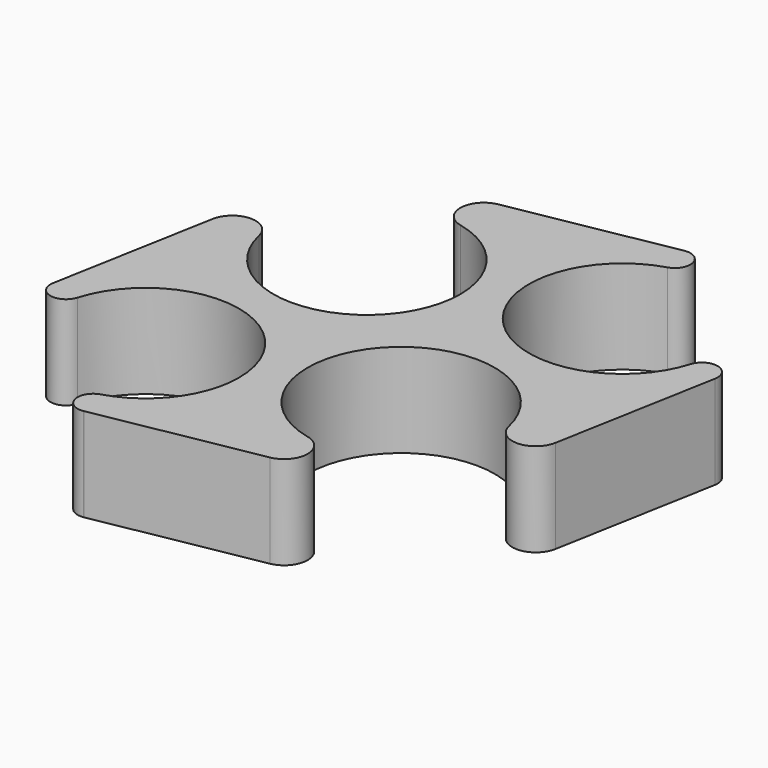
from build123d import *

# Parameters (mm, degrees)
F1_DEPTH    = 3
F2_T1_DEPTH = 13.3236108094
F2_T3_DEPTH = 16.5787171724
F3_F1_R     = 0.5
F3_F2_R     = 0.5
F3_F3_R     = 0.5
F3_F4_R     = 0.5
F4_R        = 0.75


# Not quite as in the source:
# - a fillet or chamfer that OpenCascade refuses, or shapes differently, is made with other operations: its cross-section is extruded or revolved along the edge and cut away or added


with BuildPart() as f1:
    # F0 (on Top) → F1 (new body)
    with BuildSketch(Plane.XY):
        with BuildLine():
            ThreePointArc((7.0690778624, 5.27606043), (7.204423259, 4.770944533), (7.25, 4.25))
            ThreePointArc((7.25, 4.25), (1.7925438671, 2.5292706909), (5.27606043, 7.0690778624))
            Line((5.27606043, 7.0690778624), (5.8261142664, 8.5803383574))
            Line((5.8261142664, 8.5803383574), (-4.2080450169, 6.7559457605))
            Line((-4.2080450169, 6.7559457605), (-3.77606043, 5.5690778624))
            ThreePointArc((-3.77606043, 5.5690778624), (-1.0292706909, 5.2074561329), (0.25, 2.75))
            ThreePointArc((0.25, 2.75), (-3.270944533, -0.204423259), (-5.5690778624, 3.77606043))
            Line((-5.5690778624, 3.77606043), (-6.7559457605, 4.2080450169))
            Line((-6.7559457605, 4.2080450169), (-8.5803383574, -5.8261142664))
            Line((-8.5803383574, -5.8261142664), (-7.0690778624, -5.27606043))
            ThreePointArc((-7.0690778624, -5.27606043), (-4.770944533, -1.295576741), (-1.25, -4.25))
            ThreePointArc((-1.25, -4.25), (-2.5292706909, -6.7074561329), (-5.27606043, -7.0690778624))
            Line((-5.27606043, -7.0690778624), (-5.8261142664, -8.5803383574))
            Line((-5.8261142664, -8.5803383574), (4.2080450169, -6.7559457605))
            Line((4.2080450169, -6.7559457605), (3.77606043, -5.5690778624))
            ThreePointArc((3.77606043, -5.5690778624), (0.2925438671, -1.0292706909), (5.75, -2.75))
            ThreePointArc((5.75, -2.75), (5.704423259, -3.270944533), (5.5690778624, -3.77606043))
            Line((5.5690778624, -3.77606043), (6.7559457605, -4.2080450169))
            Line((6.7559457605, -4.2080450169), (8.5803383574, 5.8261142664))
            Line((8.5803383574, 5.8261142664), (7.0690778624, 5.27606043))
        make_face()
    extrude(amount=F1_DEPTH)

    # F2: fillet of radius 2 on 8 edges, made by hand

    # F2_s2 → F2_t1 (cut)
    with BuildSketch(Plane.XY.offset(-5.1618054047)):
        with BuildLine():
            ThreePointArc((7.1252944891, -2.1766270091), (6.5910015424, -3.2135711792), (5.5690778624, -3.77606043))
            Line((5.5690778624, -3.77606043), (6.7559457605, -4.2080450169))
            Line((6.7559457605, -4.2080450169), (7.1252944891, -2.1766270091))
        make_face()
        with BuildLine():
            ThreePointArc((2.1766270091, -7.1252944891), (3.2135711792, -6.5910015424), (3.77606043, -5.5690778624))
            Line((3.77606043, -5.5690778624), (4.2080450169, -6.7559457605))
            Line((4.2080450169, -6.7559457605), (2.1766270091, -7.1252944891))
        make_face()
        with BuildLine():
            ThreePointArc((-3.77606043, 5.5690778624), (-3.2135711792, 6.5910015424), (-2.1766270091, 7.1252944891))
            Line((-2.1766270091, 7.1252944891), (-4.2080450169, 6.7559457605))
            Line((-4.2080450169, 6.7559457605), (-3.77606043, 5.5690778624))
        make_face()
        with BuildLine():
            ThreePointArc((-7.1252944891, 2.1766270091), (-6.5910015424, 3.2135711792), (-5.5690778624, 3.77606043))
            Line((-5.5690778624, 3.77606043), (-6.7559457605, 4.2080450169))
            Line((-6.7559457605, 4.2080450169), (-7.1252944891, 2.1766270091))
        make_face()
    extrude(amount=F2_T1_DEPTH, mode=Mode.SUBTRACT)

    # F2_s4 → F2_t3 (cut)
    with BuildSketch(Plane.XY.offset(-6.7893585862)):
        with BuildLine():
            ThreePointArc((7.0690778624, 5.27606043), (7.9275306923, 4.382198961), (8.0945314031, 3.1541760177))
            Line((8.0945314031, 3.1541760177), (8.5803383574, 5.8261142664))
            Line((8.5803383574, 5.8261142664), (7.0690778624, 5.27606043))
        make_face()
        with BuildLine():
            ThreePointArc((3.1541760177, 8.0945314031), (4.382198961, 7.9275306923), (5.27606043, 7.0690778624))
            Line((5.27606043, 7.0690778624), (5.8261142664, 8.5803383574))
            Line((5.8261142664, 8.5803383574), (3.1541760177, 8.0945314031))
        make_face()
        with BuildLine():
            ThreePointArc((-7.0690778624, -5.27606043), (-7.9275306923, -4.382198961), (-8.0945314031, -3.1541760177))
            Line((-8.0945314031, -3.1541760177), (-8.5803383574, -5.8261142664))
            Line((-8.5803383574, -5.8261142664), (-7.0690778624, -5.27606043))
        make_face()
        with BuildLine():
            ThreePointArc((-3.1541760177, -8.0945314031), (-4.382198961, -7.9275306923), (-5.27606043, -7.0690778624))
            Line((-5.27606043, -7.0690778624), (-5.8261142664, -8.5803383574))
            Line((-5.8261142664, -8.5803383574), (-3.1541760177, -8.0945314031))
        make_face()
    extrude(amount=F2_T3_DEPTH, mode=Mode.SUBTRACT)

    # F3: fillet of radius 0.5 on 4 edges, made by hand

    # F3_f1
    f3_f1_edges = [f1.edges().sort_by_distance(p)[0] for p in [
        (-5.27606043, -7.0690778624, 1.5),
    ]]
    fillet(f3_f1_edges, radius=F3_F1_R)

    # F3_f2
    f3_f2_edges = [f1.edges().sort_by_distance(p)[0] for p in [
        (-7.0690778624, -5.27606043, 1.5),
    ]]
    fillet(f3_f2_edges, radius=F3_F2_R)

    # F3_f3
    f3_f3_edges = [f1.edges().sort_by_distance(p)[0] for p in [
        (5.27606043, 7.0690778624, 1.5),
    ]]
    fillet(f3_f3_edges, radius=F3_F3_R)

    # F3_f4
    f3_f4_edges = [f1.edges().sort_by_distance(p)[0] for p in [
        (7.0690778624, 5.27606043, 1.5),
    ]]
    fillet(f3_f4_edges, radius=F3_F4_R)

    # F4
    f4_edges = [f1.edges().sort_by_distance(p)[0] for p in [
        (-5.569078, 3.77606, 1.5),
        (-3.77606, 5.569078, 1.5),
        (3.77606, -5.569078, 1.5),
        (5.569078, -3.77606, 1.5),
    ]]
    fillet(f4_edges, radius=F4_R)


solid = f1.part
